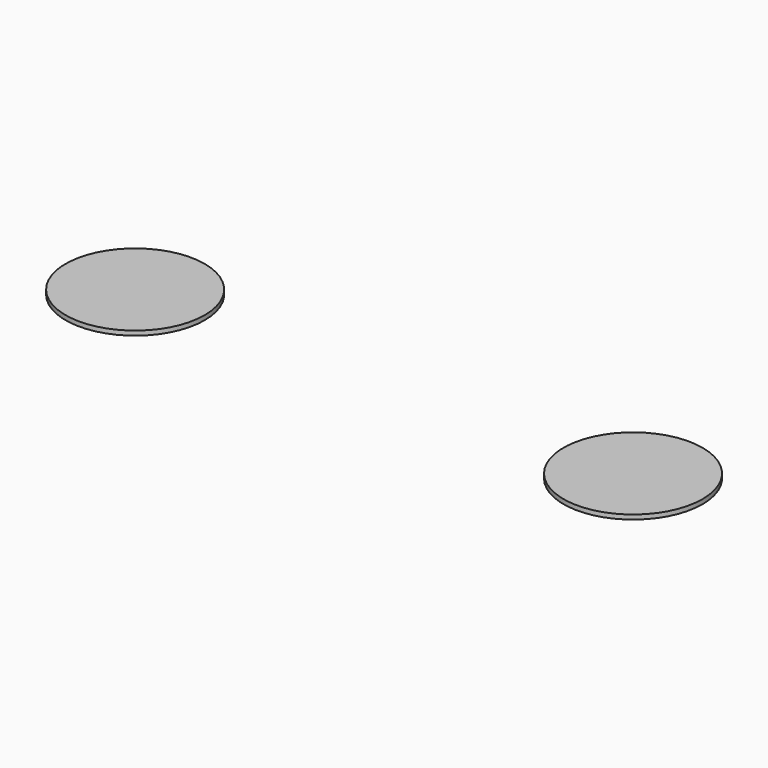
from build123d import *

# Parameters (mm, degrees)
F0_R     = 3.937
F1_DEPTH = 0.254


# Not quite as in the source:
# - the program builds the solid bodies; features that only make, move or delete a surface that nothing else refers to are left out


with BuildPart() as f1:
    # F0 (on Top) → F1 (new body)
    with BuildSketch(Plane.XY):
        with Locations((-14.6123289031, 0)):
            Circle(F0_R)
    extrude(amount=F1_DEPTH)


with BuildPart() as f1b:
    # F0 (on Top) → F1, piece 2 (new body)
    with BuildSketch(Plane.XY):
        with Locations((13.5816710969, 0)):
            Circle(F0_R)
    extrude(amount=F1_DEPTH)


solid = Compound([f1.part, f1b.part])
